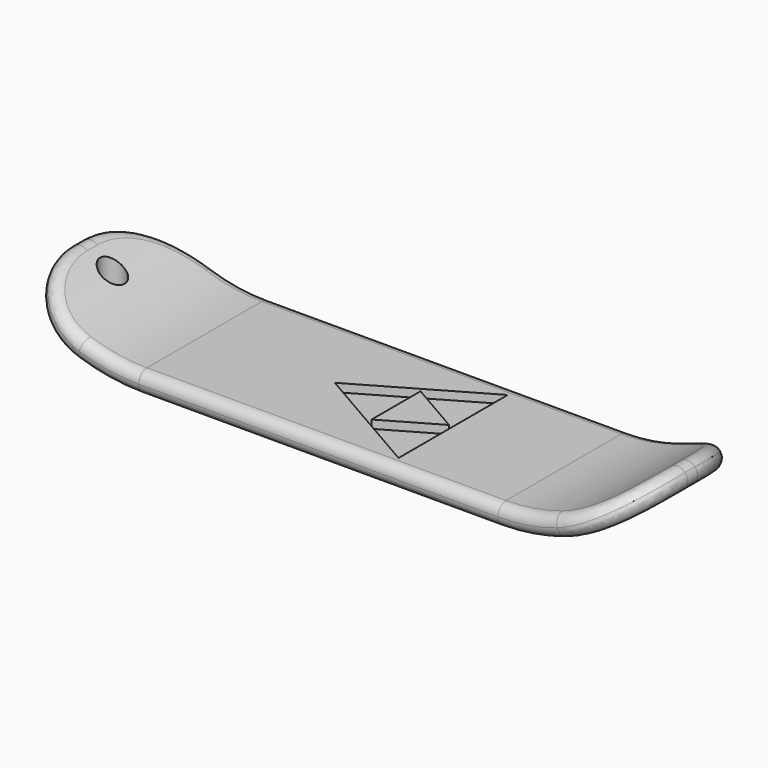
from build123d import *

# Parameters (mm, degrees)
F1_DEPTH = 10.16
F2_R     = 9.398
F3_R     = 1.2699
F4_R     = 1.524
F5_DEPTH = 25.4
F7_DEPTH = 1.016


# Not quite as in the source:
# - a fillet or chamfer is up to 0.001 mm smaller than in the source, because OpenCascade refuses the exact size


with BuildPart() as f1:
    # F0 (on Front) → F1 (new body, symmetric)
    with BuildSketch(Plane.XZ):
        with BuildLine():
            ThreePointArc((-38.735, 6.3889371363), (-31.0765340158, 1.6529325676), (-22.225, 0))
            Line((-22.225, 0), (22.225, 0))
            ThreePointArc((22.225, 0), (31.0765340158, 1.6529325676), (38.735, 6.3889371363))
            Line((38.735, 6.3889371363), (37.0252117672, 8.2672939179))
            ThreePointArc((37.0252117672, 8.2672939179), (30.1598623803, 4.0217536061), (22.225, 2.54))
            Line((22.225, 2.54), (-22.225, 2.54))
            ThreePointArc((-22.225, 2.54), (-30.1598623803, 4.0217536061), (-37.0252117672, 8.2672939179))
            Line((-37.0252117672, 8.2672939179), (-38.735, 6.3889371363))
        make_face()
    extrude(amount=F1_DEPTH, both=True)

    # F2
    f2_edges = [f1.edges().sort_by_distance(p)[0] for p in [
        (-37.880106, -10.16, 7.328116),
        (-37.880106, 10.16, 7.328116),
        (37.880106, 10.16, 7.328116),
        (37.880106, -10.16, 7.328116),
    ]]
    fillet(f2_edges, radius=F2_R)

    # F3 (radius 1.27 in the source; OpenCascade refuses exactly that, so slightly less here)
    f3_edges = [f1.edges().sort_by_distance(p)[0] for p in [
        (-25.475784, -10.16, 2.781646),
        (-36.529481, -7.486793, 4.603334),
    ]]
    fillet(f3_edges, radius=F3_R)

    # F4 (on Top) → F5 (cut)
    with BuildSketch(Plane.XY):
        with Locations((-33.6120676808, 0)):
            Circle(F4_R)
    extrude(amount=F5_DEPTH, mode=Mode.SUBTRACT)

    # F6 (on face) → F7 (cut)
    with BuildSketch(Plane.XY.offset(2.54)):
        Polygon((-6.0812620451, 0), (8.5546696342, -8.4500590949), (8.5546696342, 8.4500590949), align=None)
        Polygon((1.4907037945, -3.7850886423), (1.4907037945, 3.7850886423), (8.0466696342, 0), align=None, mode=Mode.SUBTRACT)
    extrude(amount=-F7_DEPTH, mode=Mode.SUBTRACT)


solid = f1.part
